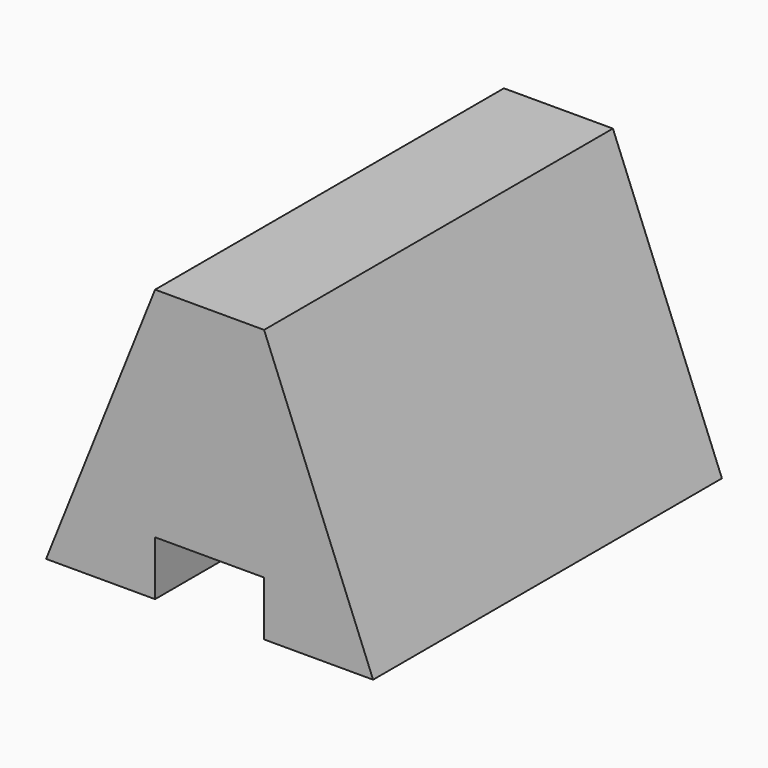
from build123d import *

# Parameters (mm, degrees)
F1_DEPTH = 25.4
F2_DEPTH = 25.4
F4_DEPTH = 50.8
F6_DEPTH = 50.8


# Not quite as in the source:
# - a feature names something its author has since deleted; it is built from what else it names


with BuildPart() as f1:
    # F0 (on Front) → F1 (new body)
    with BuildSketch(Plane.XZ):
        Polygon((-24.6924351323, 51.1944131529), (-62.7924351323, 51.1944131529), (-62.7924351323, 19.4444131529), (-50.0924351323, 19.4444131529), (-50.0924351323, 25.7944131529), (-37.3924351323, 25.7944131529), (-37.3924351323, 19.4444131529), (-24.6924351323, 19.4444131529), align=None)
    extrude(amount=F1_DEPTH)

    # F0 (on Front) + F1_face (on face) → F2 (join)
    with BuildSketch(Plane.XZ):
        Polygon((-24.6924351323, 51.1944131529), (-62.7924351323, 51.1944131529), (-62.7924351323, 19.4444131529), (-50.0924351323, 19.4444131529), (-50.0924351323, 25.7944131529), (-37.3924351323, 25.7944131529), (-37.3924351323, 19.4444131529), (-24.6924351323, 19.4444131529), align=None)
    with BuildSketch(Plane(origin=(-43.7424351323, -25.4, 36.2265560101), x_dir=(1, 0, 0), z_dir=(0, -1, 0))):
        Polygon((19.05, 14.9678571429), (-19.05, 14.9678571429), (-19.05, -16.7821428571), (-6.35, -16.7821428571), (-6.35, -10.4321428571), (6.35, -10.4321428571), (6.35, -16.7821428571), (19.05, -16.7821428571), align=None)
    extrude(amount=F2_DEPTH)

    # F3 (on face) → F4 (cut)
    with BuildSketch(Plane.XZ.offset(50.8)):
        Polygon((-62.7924351323, 19.4444131529), (-50.0924351323, 51.1944131529), (-62.7924351323, 51.1944131529), align=None)
    extrude(amount=-F4_DEPTH, mode=Mode.SUBTRACT)

    # F5 (on face) → F6 (cut)
    with BuildSketch(Plane.XZ.offset(50.8)):
        Polygon((-24.6924351323, 51.1944131529), (-37.3924351323, 51.1944131529), (-24.6924351323, 19.4444131529), align=None)
    extrude(amount=-F6_DEPTH, mode=Mode.SUBTRACT)


solid = f1.part
